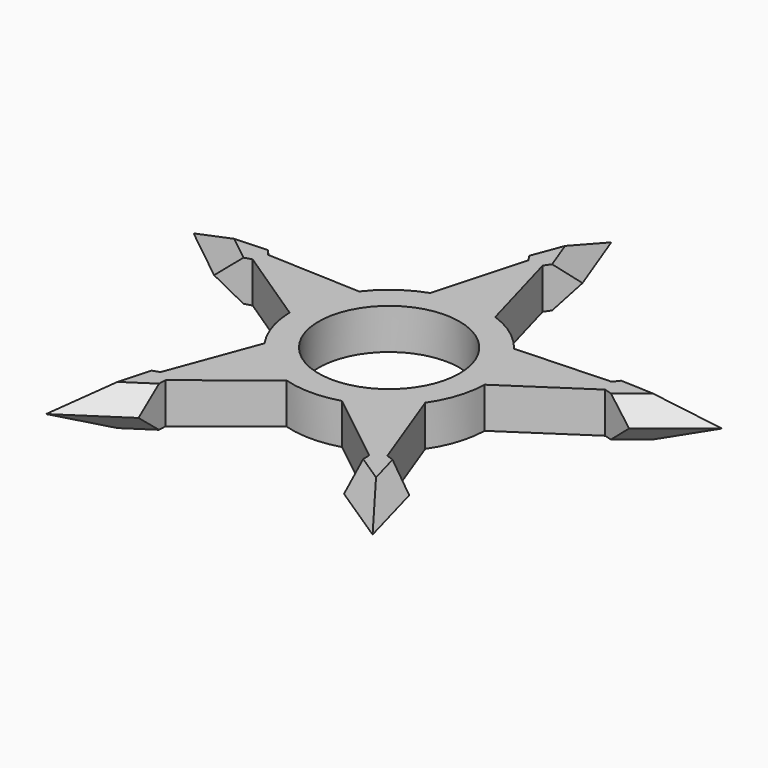
from build123d import *

# Parameters (mm, degrees)
F0_R     = 11.0000034
F1_DEPTH = 6.35
F2_SIZE  = 3.17499


# Not quite as in the source:
# - a fillet or chamfer is up to 0.001 mm smaller than in the source, because OpenCascade refuses the exact size


with BuildPart() as f1:
    # F0 (on Top) → F1 (new body)
    with BuildSketch(Plane.XY):
        with BuildLine():
            Line((-1.1111190304, 28.591448421), (-5.08, 14.3684097937))
            ThreePointArc((-5.08, 14.3684097937), (-8.9578472449, 12.3294189943), (-12.0953634317, 9.2714499112))
            Line((-12.0953634317, 9.2714499112), (-26.8487286679, 9.8919804501))
            Line((-26.8487286679, 9.8919804501), (-29.9476720311, 13.9172692636))
            Line((-29.9476720311, 13.9172692636), (-41.2574764774, 13.4053667244))
            Line((-41.2574764774, 13.4053667244), (-32.4085412404, 6.3434926108))
            Line((-32.4085412404, 6.3434926108), (-27.5354379943, 7.7785064617))
            Line((-27.5354379943, 7.7785064617), (-15.2349760945, -0.3912842944))
            ThreePointArc((-15.2349760945, -0.3912842944), (-14.4941013083, -4.7094189943), (-12.5553457071, -8.6383386236))
            Line((-12.5553457071, -8.6383386236), (-17.7045459019, -22.4778682868))
            Line((-17.7045459019, -22.4778682868), (-22.4904492218, -24.1812559153))
            Line((-22.4904492218, -24.1812559153), (-25.4985227531, -35.0957057161))
            Line((-25.4985227531, -35.0957057161), (-16.0478099898, -28.8621073099))
            Line((-16.0478099898, -28.8621073099), (-15.9067175452, -23.784067046))
            Line((-15.9067175452, -23.784067046), (-4.3357330442, -14.6102367869))
            ThreePointArc((-4.3357330442, -14.6102367869), (0, -15.24), (4.3357330442, -14.6102367869))
            Line((4.3357330442, -14.6102367869), (15.9067175452, -23.784067046))
            Line((15.9067175452, -23.784067046), (16.0478099898, -28.8621073099))
            Line((16.0478099898, -28.8621073099), (25.4985227531, -35.0957057161))
            Line((25.4985227531, -35.0957057161), (22.4904492218, -24.1812559153))
            Line((22.4904492218, -24.1812559153), (17.7045459019, -22.4778682868))
            Line((17.7045459019, -22.4778682868), (12.5553457071, -8.6383386236))
            ThreePointArc((12.5553457071, -8.6383386236), (14.4941013083, -4.7094189943), (15.2349760945, -0.3912842944))
            Line((15.2349760945, -0.3912842944), (27.5354379943, 7.7785064617))
            Line((27.5354379943, 7.7785064617), (32.4085412404, 6.3434926108))
            Line((32.4085412404, 6.3434926108), (41.2574764774, 13.4053667244))
            Line((41.2574764774, 13.4053667244), (29.9476720311, 13.9172692636))
            Line((29.9476720311, 13.9172692636), (26.8487286679, 9.8919804501))
            Line((26.8487286679, 9.8919804501), (12.0953634317, 9.2714499112))
            ThreePointArc((12.0953634317, 9.2714499112), (8.9578472449, 12.3294189943), (5.08, 14.3684097937))
            Line((5.08, 14.3684097937), (1.1111190304, 28.591448421))
            Line((1.1111190304, 28.591448421), (3.9817700226, 32.7826013508))
            Line((3.9817700226, 32.7826013508), (0, 43.3806779834))
            Line((0, 43.3806779834), (-3.9817700226, 32.7826013508))
            Line((-3.9817700226, 32.7826013508), (-1.1111190304, 28.591448421))
        make_face()
        Circle(F0_R, mode=Mode.SUBTRACT)
    extrude(amount=F1_DEPTH)

    # F2 (size 3.175 in the source; OpenCascade refuses exactly that, so slightly less here)
    f2_edges = [f1.edges().sort_by_distance(p)[0] for p in [
        (35.602574, 13.661318, 6.35),
        (35.602574, 13.661318, 0),
        (36.833009, 9.87443, 6.35),
        (36.833009, 9.87443, 0),
        (1.990885, 38.08164, 6.35),
        (1.990885, 38.08164, 0),
        (23.994486, -29.638481, 6.35),
        (23.994486, -29.638481, 0),
        (-35.602574, 13.661318, 6.35),
        (-35.602574, 13.661318, 0),
        (-1.990885, 38.08164, 6.35),
        (-1.990885, 38.08164, 0),
        (-23.994486, -29.638481, 6.35),
        (-23.994486, -29.638481, 0),
        (-36.833009, 9.87443, 6.35),
        (-36.833009, 9.87443, 0),
        (-20.773166, -31.978907, 6.35),
        (-20.773166, -31.978907, 0),
        (20.773166, -31.978907, 6.35),
        (20.773166, -31.978907, 0),
    ]]
    chamfer(f2_edges, length=F2_SIZE)


solid = f1.part
